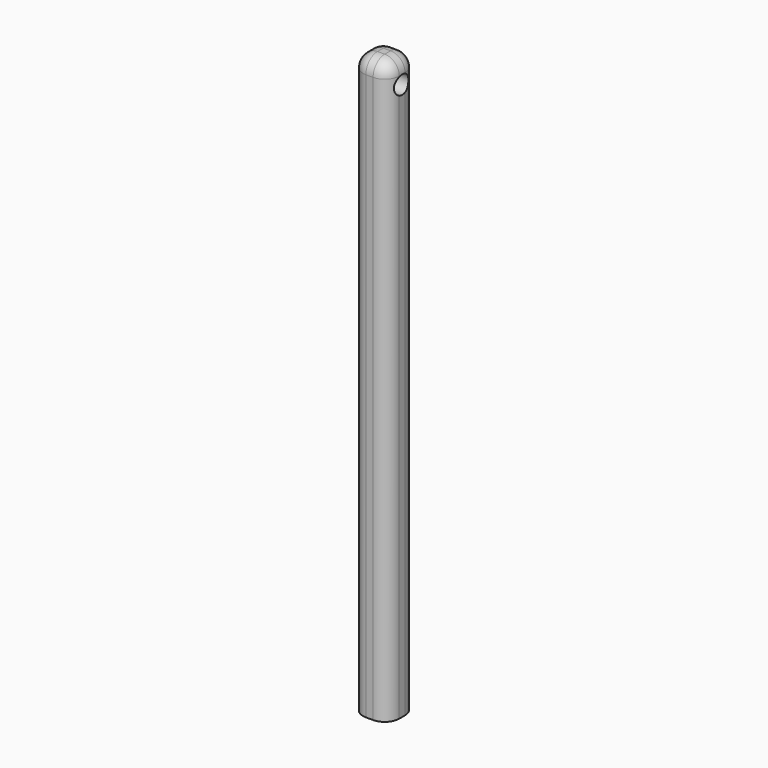
from build123d import *

# Parameters (mm, degrees)
F0_W         = 12.7
F0_H         = 12.7
F1_DEPTH     = 203.2
F2_R         = 3.175
F3_DEPTH     = 25.4
F4_T1_DEPTH  = 210.82
F4_T3_DEPTH  = 2.54
F4_T5_DEPTH  = 2.54
F4_S9_W      = 5.08
F4_S9_H      = 5.08
F4_T10_DEPTH = 5.08
F4_S15_W     = 5.08
F4_S15_H     = 5.08
F4_T16_DEPTH = 5.08
F4_S21_W     = 5.08
F4_S21_H     = 5.08
F4_T22_DEPTH = 5.08
F4_S27_W     = 5.08
F4_S27_H     = 5.08
F4_T28_DEPTH = 5.08


# Not quite as in the source:
# - a fillet or chamfer that OpenCascade refuses, or shapes differently, is made with other operations: its cross-section is extruded or revolved along the edge and cut away or added


with BuildPart() as f1:
    # F0 (on Top) → F1 (new body)
    with BuildSketch(Plane.XY):
        Rectangle(F0_W, F0_H)
    extrude(amount=F1_DEPTH)

    # F2 (on face) → F3 (cut)
    with BuildSketch(Plane.YZ.offset(6.35)):
        with Locations((0, 194.945)):
            Circle(F2_R)
    extrude(amount=-F3_DEPTH, mode=Mode.SUBTRACT)

    # F4: fillet of radius 5.08 on 8 edges, made by hand

    # F4_s2 → F4_t1 (cut)
    with BuildSketch(Plane.XY.offset(-12.7)):
        with BuildLine():
            ThreePointArc((1.27, 6.35), (4.8621024484, 4.8621024484), (6.35, 1.27))
            Line((6.35, 1.27), (6.35, 6.35))
            Line((6.35, 6.35), (1.27, 6.35))
        make_face()
        with BuildLine():
            ThreePointArc((6.35, -1.27), (4.8621024484, -4.8621024484), (1.27, -6.35))
            Line((1.27, -6.35), (6.35, -6.35))
            Line((6.35, -6.35), (6.35, -1.27))
        make_face()
        with BuildLine():
            ThreePointArc((-1.27, 6.35), (-4.8621024484, 4.8621024484), (-6.35, 1.27))
            Line((-6.35, 1.27), (-6.35, 6.35))
            Line((-6.35, 6.35), (-1.27, 6.35))
        make_face()
        with BuildLine():
            ThreePointArc((-6.35, -1.27), (-4.8621024484, -4.8621024484), (-1.27, -6.35))
            Line((-1.27, -6.35), (-6.35, -6.35))
            Line((-6.35, -6.35), (-6.35, -1.27))
        make_face()
    extrude(amount=F4_T1_DEPTH, mode=Mode.SUBTRACT)

    # F4_s4 → F4_t3 (cut)
    with BuildSketch(Plane.YZ.offset(-1.27)):
        with BuildLine():
            ThreePointArc((6.35, 198.12), (4.8621024484, 201.7121024484), (1.27, 203.2))
            Line((1.27, 203.2), (6.35, 203.2))
            Line((6.35, 203.2), (6.35, 198.12))
        make_face()
        with BuildLine():
            ThreePointArc((-1.27, 203.2), (-4.8621024484, 201.7121024484), (-6.35, 198.12))
            Line((-6.35, 198.12), (-6.35, 203.2))
            Line((-6.35, 203.2), (-1.27, 203.2))
        make_face()
    extrude(amount=F4_T3_DEPTH, mode=Mode.SUBTRACT)

    # F4_s6 → F4_t5 (cut)
    with BuildSketch(Plane.XZ.offset(-1.27)):
        with BuildLine():
            ThreePointArc((6.35, 198.12), (4.8621024484, 201.7121024484), (1.27, 203.2))
            Line((1.27, 203.2), (6.35, 203.2))
            Line((6.35, 203.2), (6.35, 198.12))
        make_face()
        with BuildLine():
            ThreePointArc((-6.35, 198.12), (-4.8621024484, 201.7121024484), (-1.27, 203.2))
            Line((-1.27, 203.2), (-6.35, 203.2))
            Line((-6.35, 203.2), (-6.35, 198.12))
        make_face()
    extrude(amount=F4_T5_DEPTH, mode=Mode.SUBTRACT)


with BuildPart() as f4_tool8:
    # F4_s9 → F4_t10 (new body)
    with BuildSketch(Plane.XZ.offset(-1.27)):
        with Locations((3.81, 200.66)):
            Rectangle(F4_S9_W, F4_S9_H)
    extrude(amount=-F4_T10_DEPTH)

    # F4_s11 → F4_t12 (revolve, cut)
    with BuildSketch(Plane(origin=(1.27, 1.27, 198.12), x_dir=(-0.7071067812, 0, -0.7071067812), z_dir=(0.7071067812, 0, -0.7071067812))):
        with BuildLine():
            ThreePointArc((0, -5.08), (5.08, 0), (0, 5.08))
            Line((0, 5.08), (0, -5.08))
        make_face()
    revolve(axis=Axis((1.27, 1.27, 198.12), (0, 1, 0)), mode=Mode.SUBTRACT)


with BuildPart() as f1_1:
    add(f1.part)

    # F4_t7: cut F4_tool8
    add(f4_tool8.part, mode=Mode.SUBTRACT)


with BuildPart() as f4_tool14:
    # F4_s15 → F4_t16 (new body)
    with BuildSketch(Plane.YZ.offset(1.27)):
        with Locations((-3.81, 200.66)):
            Rectangle(F4_S15_W, F4_S15_H)
    extrude(amount=F4_T16_DEPTH)

    # F4_s17 → F4_t18 (revolve, cut)
    with BuildSketch(Plane(origin=(1.27, -1.27, 198.12), x_dir=(0, 0.7071067812, -0.7071067812), z_dir=(0, -0.7071067812, -0.7071067812))):
        with BuildLine():
            ThreePointArc((0, -5.08), (5.08, 0), (0, 5.08))
            Line((0, 5.08), (0, -5.08))
        make_face()
    revolve(axis=Axis((1.27, -1.27, 198.12), (1, 0, 0)), mode=Mode.SUBTRACT)


with BuildPart() as f1_2:
    add(f1_1.part)

    # F4_t13: cut F4_tool14
    add(f4_tool14.part, mode=Mode.SUBTRACT)


with BuildPart() as f4_tool20:
    # F4_s21 → F4_t22 (new body)
    with BuildSketch(Plane.XZ.offset(-1.27)):
        with Locations((-3.81, 200.66)):
            Rectangle(F4_S21_W, F4_S21_H)
    extrude(amount=-F4_T22_DEPTH)

    # F4_s23 → F4_t24 (revolve, cut)
    with BuildSketch(Plane(origin=(-1.27, 1.27, 198.12), x_dir=(0.7071067812, 0, -0.7071067812), z_dir=(0.7071067812, 0, 0.7071067812))):
        with BuildLine():
            ThreePointArc((0, -5.08), (5.08, 0), (0, 5.08))
            Line((0, 5.08), (0, -5.08))
        make_face()
    revolve(axis=Axis((-1.27, 1.27, 198.12), (0, 1, 0)), mode=Mode.SUBTRACT)


with BuildPart() as f1_3:
    add(f1_2.part)

    # F4_t19: cut F4_tool20
    add(f4_tool20.part, mode=Mode.SUBTRACT)


with BuildPart() as f4_tool26:
    # F4_s27 → F4_t28 (new body)
    with BuildSketch(Plane.YZ.offset(-1.27)):
        with Locations((-3.81, 200.66)):
            Rectangle(F4_S27_W, F4_S27_H)
    extrude(amount=-F4_T28_DEPTH)

    # F4_s29 → F4_t30 (revolve, cut)
    with BuildSketch(Plane(origin=(-1.27, -1.27, 198.12), x_dir=(0, 0.7071067812, -0.7071067812), z_dir=(0, 0.7071067812, 0.7071067812))):
        with BuildLine():
            ThreePointArc((0, -5.08), (5.08, 0), (0, 5.08))
            Line((0, 5.08), (0, -5.08))
        make_face()
    revolve(axis=Axis((-1.27, -1.27, 198.12), (-1, 0, 0)), mode=Mode.SUBTRACT)


with BuildPart() as f1_4:
    add(f1_3.part)

    # F4_t25: cut F4_tool26
    add(f4_tool26.part, mode=Mode.SUBTRACT)


solid = f1_4.part
